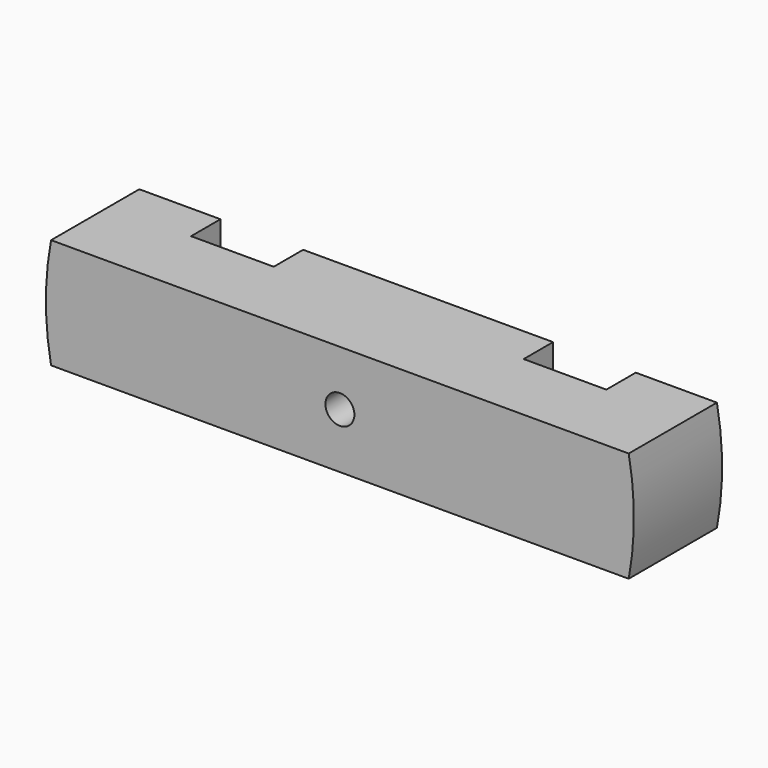
from build123d import *

# Parameters (mm, degrees)
F1_DEPTH = 3.81
F2_R     = 0.5
F3_DEPTH = 25.4
F5_DEPTH = 1.27


# Not quite as in the source:
# - ends of sketch curves that miss each other by under 0.0002 mm in the source are joined


with BuildPart() as f1:
    # F0 (on Front) → F1 (new body)
    with BuildSketch(Plane.XZ):
        with BuildLine():
            Line((9.9798112172, 1.905), (-9.9798084652, 1.905))
            ThreePointArc((-9.9798084652, 1.905), (-10.16, 0), (-9.9798084652, -1.9049994747))
            Line((-9.9798084652, -1.9049994747), (9.9798084652, -1.905))
            ThreePointArc((9.9798084652, -1.905), (10.16, 0), (9.9798112172, 1.905))
        make_face()
    extrude(amount=F1_DEPTH)

    # F2 (on face) → F3 (cut)
    with BuildSketch(Plane.XZ.offset(3.81)):
        Circle(F2_R)
    extrude(amount=-F3_DEPTH, mode=Mode.SUBTRACT)

    # F4 (on face) → F5 (cut)
    with BuildSketch(Plane.XZ):
        Polygon((7.1755, 1.905), (4.318, 1.905), (4.318, -0.0512809254), (4.318, -1.905), (7.1755, -1.905), align=None)
        Polygon((-4.318, 0), (-4.318, 1.905), (-7.1755, 1.905), (-7.1755, -1.905), (-4.318, -1.905), align=None)
    extrude(amount=F5_DEPTH, mode=Mode.SUBTRACT)


solid = f1.part
